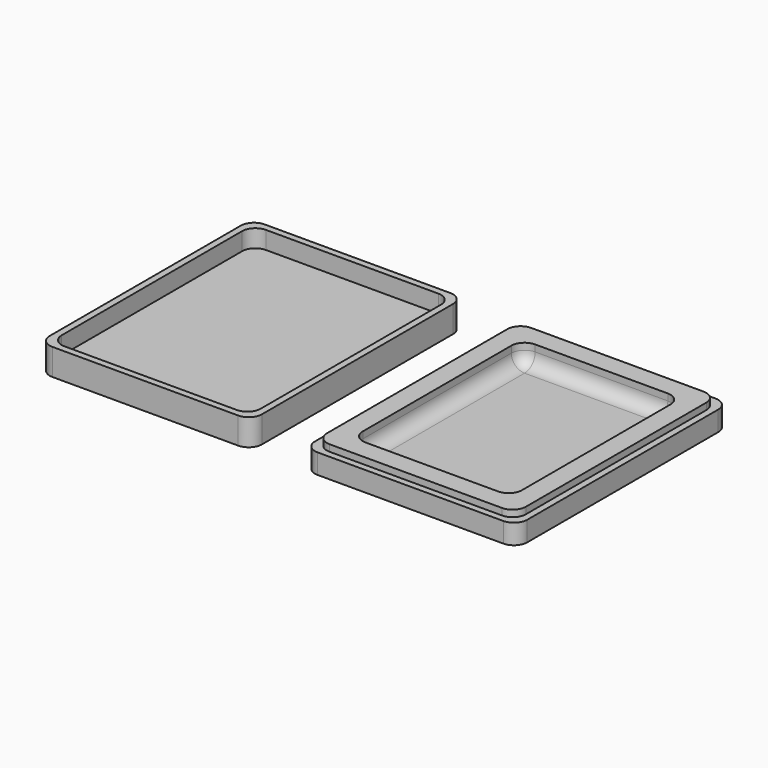
from build123d import *

# Parameters (mm, degrees)
F2_W     = 101.6
F2_H     = 127
F2_W_2   = 95.25
F2_H_2   = 120.65
F3_DEPTH = 9.525
F2_W_3   = 76.2
F2_H_3   = 101.6
F4_DEPTH = 3.175
F5_DEPTH = 12.7
F7_DEPTH = 4.2333333333
F8_DEPTH = 12.7
F10_R    = 6.35
F11_R    = 6.35


# Not quite as in the source:
# - a variable given as a bare number and used for a length is read in inches; the dataset says mm whatever the document's units were


with BuildPart() as f3:
    # F2 (on Top) → F3 (new body)
    with BuildSketch(Plane.XY):
        Rectangle(F2_W, F2_H)
        Rectangle(F2_W_2, F2_H_2, mode=Mode.SUBTRACT)
    extrude(amount=F3_DEPTH)



with BuildPart() as f4:
    # F2 (on Top) → F4 (new body)
    with BuildSketch(Plane.XY):
        Rectangle(F2_W_3, F2_H_3)
    extrude(amount=F4_DEPTH)


with BuildPart() as f3_1:
    add(f3.part)

    add(f4.part)  # F5 merges F4
    # F2 (on Top) → F5 (join)
    with BuildSketch(Plane.XY):
        Rectangle(F2_W_2, F2_H_2)
        Rectangle(F2_W_3, F2_H_3, mode=Mode.SUBTRACT)
    extrude(amount=F5_DEPTH)


with BuildPart() as f3_2:
    # F6: moved
    add(f3_1.part.moved(Location((127, 0, 0))))

    # F10
    f10_edges = [f3_2.edges().sort_by_distance(p)[0] for p in [
        (177.8, -63.5, 4.7625),
        (174.625, -60.325, 11.1125),
        (165.1, -50.8, 7.9375),
        (76.2, -63.5, 4.7625),
        (79.375, -60.325, 11.1125),
        (88.9, -50.8, 7.9375),
        (76.2, 63.5, 4.7625),
        (79.375, 60.325, 11.1125),
        (88.9, 50.8, 7.9375),
        (177.8, 63.5, 4.7625),
        (174.625, 60.325, 11.1125),
        (165.1, 50.8, 7.9375),
        (127, 50.8, 3.175),
        (165.1, 0, 3.175),
        (88.9, 0, 3.175),
        (127, -50.8, 3.175),
    ]]
    fillet(f10_edges, radius=F10_R)


with BuildPart() as f7:
    # F2 (on Top) → F7 (new body)
    with BuildSketch(Plane.XY):
        Rectangle(F2_W_2, F2_H_2)
        Rectangle(F2_W_3, F2_H_3, mode=Mode.SUBTRACT)
        Rectangle(F2_W_3, F2_H_3)
    extrude(amount=F7_DEPTH)

    # F2 (on Top) → F8 (join)
    with BuildSketch(Plane.XY):
        Rectangle(F2_W, F2_H)
        Rectangle(F2_W_2, F2_H_2, mode=Mode.SUBTRACT)
    extrude(amount=F8_DEPTH)

    # F11
    f11_edges = [f7.edges().sort_by_distance(p)[0] for p in [
        (50.8, 63.5, 6.35),
        (47.625, 60.325, 8.466667),
        (-50.8, 63.5, 6.35),
        (-47.625, 60.325, 8.466667),
        (-50.8, -63.5, 6.35),
        (-47.625, -60.325, 8.466667),
        (47.625, -60.325, 8.466667),
        (50.8, -63.5, 6.35),
    ]]
    fillet(f11_edges, radius=F11_R)


solid = Compound([f3_2.part, f7.part])
